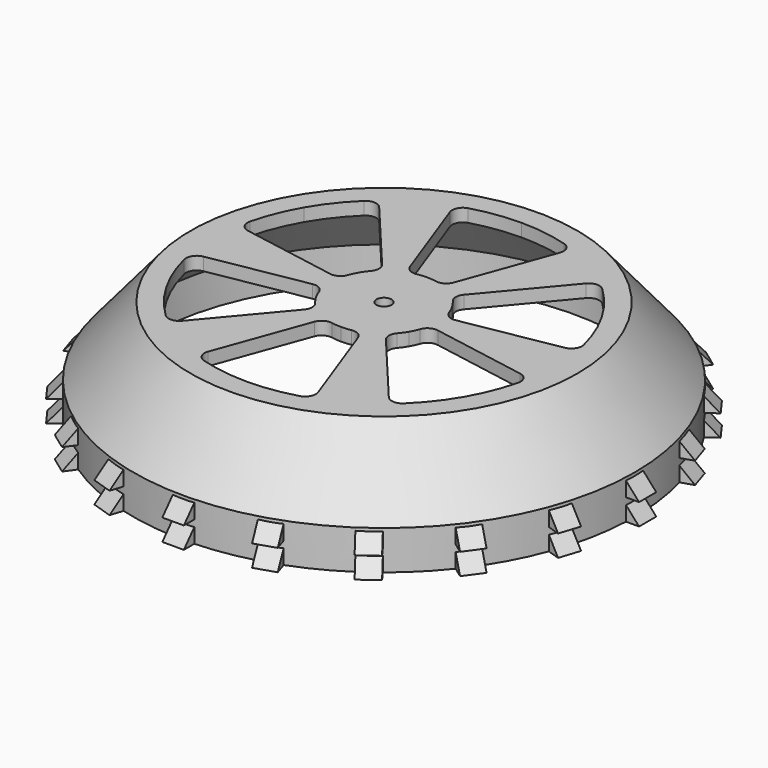
from build123d import *

# Parameters (mm, degrees)
F2_R            = 3.5
F3_DEPTH        = 25
F5_DEPTH        = 25
F5_COPIES_COUNT = 6
F6_R            = 5
F8_DEPTH        = 5
F8_COPIES_COUNT = 20


# Not quite as in the source:
# - a pattern or mirror of a feature is missing from the dataset's text; its kind, count and spacing are read off the source's solid


with BuildPart() as f1:
    # F0 (on Front) → F1 (revolve)
    with BuildSketch(Plane.XZ):
        Polygon((90, 0), (0, 0), (0, -6), (87.2021540511, -6), (110.6924196096, -33.9946083704), (110.6924196096, -50), (116.6924196096, -50), (116.6924196096, -31.8107869648), align=None)
    revolve(axis=Axis((0, 0, -3), (0, 0, -1)))

    # F2 (on face) → F3 (cut)
    with BuildSketch(Plane.XY):
        Circle(F2_R)
    extrude(amount=-F3_DEPTH, mode=Mode.SUBTRACT)

    # F4 (on face) → F5 (cut)
    with BuildSketch(Plane.XY):
        with BuildLine():
            Line((-27.3616114661, 75.1754096629), (-8.5505035831, 23.4923155196))
            ThreePointArc((-8.5505035831, 23.4923155196), (-4.3412044417, 24.6201938253), (0, 25))
            ThreePointArc((0, 25), (4.3412044417, 24.6201938253), (8.5505035831, 23.4923155196))
            Line((8.5505035831, 23.4923155196), (27.3616114661, 75.1754096629))
            ThreePointArc((27.3616114661, 75.1754096629), (13.8918542134, 78.784620241), (0, 80))
            ThreePointArc((0, 80), (-13.8918542134, 78.784620241), (-27.3616114661, 75.1754096629))
        make_face()
    f5 = extrude(amount=-F5_DEPTH, mode=Mode.SUBTRACT)

    # F5_copies: F5 ×6 about axis
    f5_copies_axis = Axis((0, 0, 0), (0, 0, 1))
    for i in range(1, F5_COPIES_COUNT):
        add(f5.rotate(f5_copies_axis, i * 360 / F5_COPIES_COUNT), mode=Mode.SUBTRACT)

    # F6
    f6_edges = [f1.edges().sort_by_distance(p)[0] for p in [
        (8.550504, 23.492316, -3),
        (-8.550504, 23.492316, -3),
        (27.361611, 75.17541, -3),
        (-27.361611, 75.17541, -3),
        (-78.78462, 13.891854, -3),
        (-51.423009, 61.283555, -3),
        (-24.620194, 4.341204, -3),
        (-16.06969, 19.151111, -3),
        (51.423009, 61.283555, -3),
        (78.78462, 13.891854, -3),
        (24.620194, 4.341204, -3),
        (16.06969, 19.151111, -3),
        (-51.423009, -61.283555, -3),
        (-78.78462, -13.891854, -3),
        (-16.06969, -19.151111, -3),
        (-24.620194, -4.341204, -3),
        (27.361611, -75.17541, -3),
        (-27.361611, -75.17541, -3),
        (8.550504, -23.492316, -3),
        (-8.550504, -23.492316, -3),
        (78.78462, -13.891854, -3),
        (51.423009, -61.283555, -3),
        (24.620194, -4.341204, -3),
        (16.06969, -19.151111, -3),
    ]]
    fillet(f6_edges, radius=F6_R)

    # F7 (on Front) → F8 (join, symmetric)
    with BuildSketch(Plane.XZ):
        Polygon((-122.6924196096, -50), (-114.6924196096, -50), (-114.6924196096, -41), align=None)
        Polygon((-122.6924196096, -40), (-114.6924196096, -40), (-114.6924196096, -31), align=None)
    f8 = extrude(amount=F8_DEPTH, both=True)

    # F8_copies: F8 ×20 about axis
    f8_copies_axis = Axis((0, 0, 0), (0, 0, 1))
    for i in range(1, F8_COPIES_COUNT):
        add(f8.rotate(f8_copies_axis, i * 360 / F8_COPIES_COUNT))


solid = f1.part
